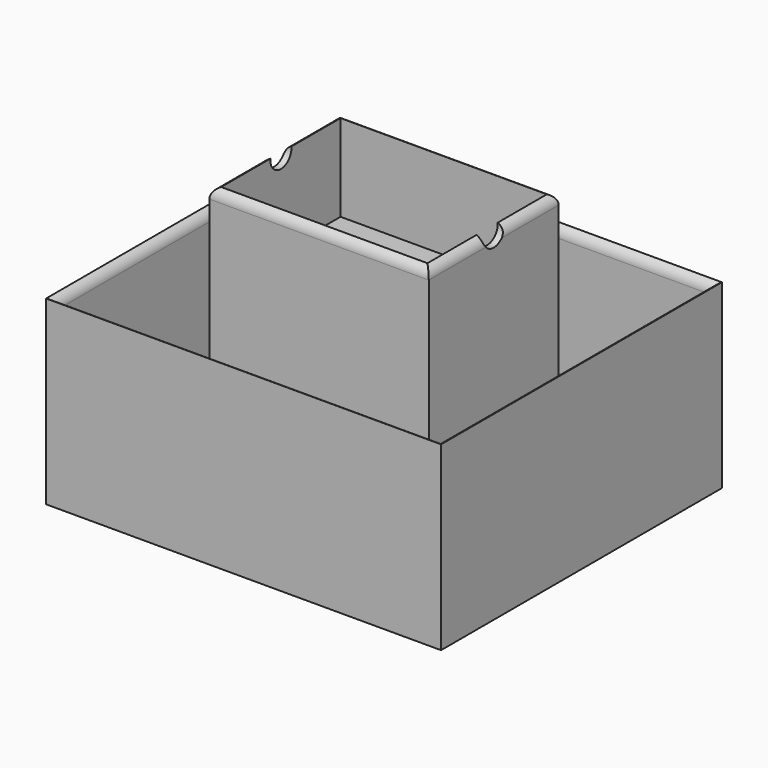
from build123d import *

# Parameters (mm, degrees)
F0_W          = 180
F0_H          = 160
F1_DEPTH      = 1
F2_W          = 10
F2_H          = 10
F3_DEPTH      = 50
F4_T          = 1
F4_T3_DEPTH   = 12
F4_T5_DEPTH   = 12
F4_T7_DEPTH   = 12
F4_T9_DEPTH   = 12
F5_W          = 180
F5_H          = 160
F6_DEPTH      = 3
F7_W          = 180
F7_H          = 160
F7_W_2        = 174
F7_H_2        = 154
F8_DEPTH      = 80
F9_W          = 100
F9_H          = 74
F10_DEPTH     = 120
F11_W         = 94
F11_H         = 68
F12_DEPTH     = 40
F14_T1_DEPTH  = 125
F14_T3_DEPTH  = 99
F14_T5_DEPTH  = 174
F14_T7_DEPTH  = 154
F14_T13_DEPTH = 166.5
F14_T19_DEPTH = 186.5
F14_T28_DEPTH = 166.5
F14_T34_DEPTH = 186.5
F14_T43_DEPTH = 186.5
F14_T49_DEPTH = 166.5
F14_T58_DEPTH = 166.5
F14_T64_DEPTH = 186.5
F15_R         = 6.0326848408
F16_DEPTH     = 500
F17_W         = 180
F17_H         = 160
F18_DEPTH     = 51
F13_W         = 94
F13_H         = 68
F19_DEPTH     = 80


# Not quite as in the source:
# - a fillet or chamfer that OpenCascade refuses, or shapes differently, is made with other operations: its cross-section is extruded or revolved along the edge and cut away or added
# - a shell that OpenCascade refuses in one call is made with other operations: the cavity is built on its own and cut out


with BuildPart() as f1:
    # F0 (on Top) → F1 (new body)
    with BuildSketch(Plane.XY):
        with Locations((-40, 0)):
            Rectangle(F0_W, F0_H)
    extrude(amount=F1_DEPTH)

    # F2 (on face) → F3 (join)
    with BuildSketch(Plane.XY.offset(1)):
        with Locations((-125, 75)):
            Rectangle(F2_W, F2_H)
        with Locations((45, 75)):
            Rectangle(F2_W, F2_H)
        with Locations((-125, -75)):
            Rectangle(F2_W, F2_H)
        with Locations((45, -75)):
            Rectangle(F2_W, F2_H)
    extrude(amount=F3_DEPTH)

    # F4: shell of thickness 1, made by hand


with BuildPart() as f4_core1:
    # F4_t2: copy of F1
    add(f1.part)

    # the walls: a layer under each face that stays
    f4_faces = [f4_core1.faces().sort_by_distance(p)[0] for p in [
        (44, 80, 49.3),
        (-124, -80, 49.3),
        (45, -75, 51),
        (45, -70, 26),
        (40, -75, 26),
        (-120, -75, 26),
        (-125, -70, 26),
        (-125, -75, 51),
        (-130, 74.6666666667, 49.3),
        (-125, 70, 26),
        (-125, 75, 51),
        (-120, 75, 26),
        (-40, 0, 1),
        (45, 70, 26),
        (40, 75, 26),
        (45, 75, 51),
        (50, -74.6666666667, 49.3),
    ]]
    thicken(f4_faces, amount=-F4_T, mode=Mode.SUBTRACT)

    # F4_s4 → F4_t3 (cut)
    with BuildSketch(Plane.YZ.offset(39)):
        Polygon((-69.99, 1.01), (-71, 1), (-71, 0), (-70, 0), align=None)
        Polygon((69.99, 1.01), (70, 0), (71, 0), (71, 1), align=None)
    extrude(amount=F4_T3_DEPTH, mode=Mode.SUBTRACT)

    # F4_s6 → F4_t5 (cut)
    with BuildSketch(Plane.XZ.offset(69)):
        Polygon((39.99, 1.01), (41, 1), (41, 0), (40, 0), align=None)
        Polygon((-119.99, 1.01), (-121, 1), (-121, 0), (-120, 0), align=None)
    extrude(amount=F4_T5_DEPTH, mode=Mode.SUBTRACT)

    # F4_s8 → F4_t7 (cut)
    with BuildSketch(Plane.YZ.offset(-131)):
        Polygon((-69.99, 1.01), (-71, 1), (-71, 0), (-70, 0), align=None)
        Polygon((69.99, 1.01), (71, 1), (71, 0), (70, 0), align=None)
    extrude(amount=F4_T7_DEPTH, mode=Mode.SUBTRACT)

    # F4_s10 → F4_t9 (cut)
    with BuildSketch(Plane.XZ.offset(-81)):
        Polygon((-119.99, 1.01), (-121, 1), (-121, 0), (-120, 0), align=None)
        Polygon((39.99, 1.01), (40, 0), (41, 0), (41, 1), align=None)
    extrude(amount=F4_T9_DEPTH, mode=Mode.SUBTRACT)


with BuildPart() as f1_1:
    add(f1.part)

    # what is left inside the walls is the cavity
    f4_cavity = [f4_core1.part.solids().sort_by_distance(p)[0] for p in [
        (45, 78.99, 33.333333),
        (-125, 78.99, 33.333333),
        (48.99, -75, 33.333333),
        (-123.666667, -71.01, 25),
    ]]
    add(f4_cavity, mode=Mode.SUBTRACT)

    # F5 (on face) → F6 (join)
    with BuildSketch(Plane.XY.offset(51)):
        with Locations((-40, 0)):
            Rectangle(F5_W, F5_H)
    extrude(amount=F6_DEPTH)

    # F7 (on face) → F8 (join)
    with BuildSketch(Plane.XY.offset(54)):
        with Locations((-40, 0)):
            Rectangle(F7_W, F7_H)
        with Locations((-40, 0)):
            Rectangle(F7_W_2, F7_H_2, mode=Mode.SUBTRACT)
    extrude(amount=F8_DEPTH)

    # F9 (on face) → F10 (join)
    with BuildSketch(Plane.XY.offset(54)):
        with Locations((-40, 0)):
            Rectangle(F9_W, F9_H)
    extrude(amount=F10_DEPTH)

    # F11 (on face) → F12 (cut)
    with BuildSketch(Plane.XY.offset(174)):
        with Locations((-40, 0)):
            Rectangle(F11_W, F11_H)
    extrude(amount=-F12_DEPTH, mode=Mode.SUBTRACT)

    # F14: fillet of radius 5 on 8 edges, made by hand

    # F14_s2 → F14_t1 (cut)
    with BuildSketch(Plane.YZ.offset(-102.5)):
        with BuildLine():
            ThreePointArc((-37, 169), (-35.5355339059, 172.5355339059), (-32, 174))
            Line((-32, 174), (-37, 174))
            Line((-37, 174), (-37, 169))
        make_face()
        with BuildLine():
            ThreePointArc((37, 169), (35.5355339059, 172.5355339059), (32, 174))
            Line((32, 174), (37, 174))
            Line((37, 174), (37, 169))
        make_face()
    extrude(amount=F14_T1_DEPTH, mode=Mode.SUBTRACT)

    # F14_s4 → F14_t3 (cut)
    with BuildSketch(Plane.XZ.offset(-49.5)):
        with BuildLine():
            ThreePointArc((-90, 169), (-88.5355339059, 172.5355339059), (-85, 174))
            Line((-85, 174), (-90, 174))
            Line((-90, 174), (-90, 169))
        make_face()
        with BuildLine():
            ThreePointArc((10, 169), (8.5355339059, 172.5355339059), (5, 174))
            Line((5, 174), (10, 174))
            Line((10, 174), (10, 169))
        make_face()
    extrude(amount=F14_T3_DEPTH, mode=Mode.SUBTRACT)

    # F14_s6 → F14_t5 (cut)
    with BuildSketch(Plane.YZ.offset(-127)):
        with BuildLine():
            ThreePointArc((-82, 134), (-78.4644660941, 132.5355339059), (-77, 129))
            Line((-77, 129), (-77, 134))
            Line((-77, 134), (-82, 134))
        make_face()
        with BuildLine():
            ThreePointArc((82, 134), (78.4644660941, 132.5355339059), (77, 129))
            Line((77, 129), (77, 134))
            Line((77, 134), (82, 134))
        make_face()
    extrude(amount=F14_T5_DEPTH, mode=Mode.SUBTRACT)

    # F14_s8 → F14_t7 (cut)
    with BuildSketch(Plane.XZ.offset(-77)):
        with BuildLine():
            ThreePointArc((52, 134), (48.4644660941, 132.5355339059), (47, 129))
            Line((47, 129), (47, 134))
            Line((47, 134), (52, 134))
        make_face()
        with BuildLine():
            ThreePointArc((-132, 134), (-128.4644660941, 132.5355339059), (-127, 129))
            Line((-127, 129), (-127, 134))
            Line((-127, 134), (-132, 134))
        make_face()
    extrude(amount=F14_T7_DEPTH, mode=Mode.SUBTRACT)


with BuildPart() as f14_tool11:
    # F14_s12 → F14_t13 (new body)
    with BuildSketch(Plane.XZ.offset(-77)):
        with BuildLine():
            ThreePointArc((52, 134), (48.4644660941, 132.5355339059), (47, 129))
            Line((47, 129), (47, 134))
            Line((47, 134), (52, 134))
        make_face()
    extrude(amount=F14_T13_DEPTH)

    split(bisect_by=Plane.YZ.offset(50), keep=Keep.BOTTOM)

    split(bisect_by=Plane.XZ.offset(80), keep=Keep.BOTTOM)

    split(bisect_by=Plane.XZ.offset(77), keep=Keep.TOP)


with BuildPart() as f14_tool17:
    # F14_s18 → F14_t19 (new body)
    with BuildSketch(Plane.YZ.offset(59.5)):
        with BuildLine():
            ThreePointArc((-82, 134), (-78.4644660941, 132.5355339059), (-77, 129))
            Line((-77, 129), (-77, 134))
            Line((-77, 134), (-82, 134))
        make_face()
    extrude(amount=-F14_T19_DEPTH)

    split(bisect_by=Plane.YZ.offset(50), keep=Keep.BOTTOM)

    split(bisect_by=Plane.XZ.offset(80), keep=Keep.BOTTOM)

    split(bisect_by=Plane.YZ.offset(47), keep=Keep.TOP)


with BuildPart() as f14_tool11_1:
    add(f14_tool11.part)

    # F14_t23: intersect F14_tool17
    add(f14_tool17.part, mode=Mode.INTERSECT)


with BuildPart() as f1_2:
    add(f1_1.part)

    # F14_t9: cut F14_tool11
    add(f14_tool11_1.part, mode=Mode.SUBTRACT)


with BuildPart() as f14_tool26:
    # F14_s27 → F14_t28 (new body)
    with BuildSketch(Plane.XZ.offset(89.5)):
        with BuildLine():
            ThreePointArc((-132, 134), (-128.4644660941, 132.5355339059), (-127, 129))
            Line((-127, 129), (-127, 134))
            Line((-127, 134), (-132, 134))
        make_face()
    extrude(amount=-F14_T28_DEPTH)

    split(bisect_by=Plane.YZ.offset(-130), keep=Keep.TOP)

    split(bisect_by=Plane.XZ.offset(80), keep=Keep.BOTTOM)

    split(bisect_by=Plane.XZ.offset(77), keep=Keep.TOP)


with BuildPart() as f14_tool32:
    # F14_s33 → F14_t34 (new body)
    with BuildSketch(Plane.YZ.offset(47)):
        with BuildLine():
            ThreePointArc((-82, 134), (-78.4644660941, 132.5355339059), (-77, 129))
            Line((-77, 129), (-77, 134))
            Line((-77, 134), (-82, 134))
        make_face()
    extrude(amount=-F14_T34_DEPTH)

    split(bisect_by=Plane.YZ.offset(-130), keep=Keep.TOP)

    split(bisect_by=Plane.XZ.offset(80), keep=Keep.BOTTOM)

    split(bisect_by=Plane.YZ.offset(-127), keep=Keep.BOTTOM)


with BuildPart() as f14_tool26_1:
    add(f14_tool26.part)

    # F14_t38: intersect F14_tool32
    add(f14_tool32.part, mode=Mode.INTERSECT)


with BuildPart() as f1_3:
    add(f1_2.part)

    # F14_t24: cut F14_tool26
    add(f14_tool26_1.part, mode=Mode.SUBTRACT)


with BuildPart() as f14_tool41:
    # F14_s42 → F14_t43 (new body)
    with BuildSketch(Plane.YZ.offset(-127)):
        with BuildLine():
            ThreePointArc((82, 134), (78.4644660941, 132.5355339059), (77, 129))
            Line((77, 129), (77, 134))
            Line((77, 134), (82, 134))
        make_face()
    extrude(amount=F14_T43_DEPTH)

    split(bisect_by=Plane.XZ.offset(-80), keep=Keep.TOP)

    split(bisect_by=Plane.YZ.offset(50), keep=Keep.BOTTOM)

    split(bisect_by=Plane.YZ.offset(47), keep=Keep.TOP)


with BuildPart() as f14_tool47:
    # F14_s48 → F14_t49 (new body)
    with BuildSketch(Plane.XZ.offset(-89.5)):
        with BuildLine():
            ThreePointArc((52, 134), (48.4644660941, 132.5355339059), (47, 129))
            Line((47, 129), (47, 134))
            Line((47, 134), (52, 134))
        make_face()
    extrude(amount=F14_T49_DEPTH)

    split(bisect_by=Plane.XZ.offset(-80), keep=Keep.TOP)

    split(bisect_by=Plane.YZ.offset(50), keep=Keep.BOTTOM)

    split(bisect_by=Plane.XZ.offset(-77), keep=Keep.BOTTOM)


with BuildPart() as f14_tool41_1:
    add(f14_tool41.part)

    # F14_t53: intersect F14_tool47
    add(f14_tool47.part, mode=Mode.INTERSECT)


with BuildPart() as f1_4:
    add(f1_3.part)

    # F14_t39: cut F14_tool41
    add(f14_tool41_1.part, mode=Mode.SUBTRACT)


with BuildPart() as f14_tool56:
    # F14_s57 → F14_t58 (new body)
    with BuildSketch(Plane.XZ.offset(77)):
        with BuildLine():
            ThreePointArc((-132, 134), (-128.4644660941, 132.5355339059), (-127, 129))
            Line((-127, 129), (-127, 134))
            Line((-127, 134), (-132, 134))
        make_face()
    extrude(amount=-F14_T58_DEPTH)

    split(bisect_by=Plane.XZ.offset(-80), keep=Keep.TOP)

    split(bisect_by=Plane.YZ.offset(-130), keep=Keep.TOP)

    split(bisect_by=Plane.XZ.offset(-77), keep=Keep.BOTTOM)


with BuildPart() as f14_tool62:
    # F14_s63 → F14_t64 (new body)
    with BuildSketch(Plane.YZ.offset(-139.5)):
        with BuildLine():
            ThreePointArc((82, 134), (78.4644660941, 132.5355339059), (77, 129))
            Line((77, 129), (77, 134))
            Line((77, 134), (82, 134))
        make_face()
    extrude(amount=F14_T64_DEPTH)

    split(bisect_by=Plane.XZ.offset(-80), keep=Keep.TOP)

    split(bisect_by=Plane.YZ.offset(-130), keep=Keep.TOP)

    split(bisect_by=Plane.YZ.offset(-127), keep=Keep.BOTTOM)


with BuildPart() as f14_tool56_1:
    add(f14_tool56.part)

    # F14_t68: intersect F14_tool62
    add(f14_tool62.part, mode=Mode.INTERSECT)


with BuildPart() as f1_5:
    add(f1_4.part)

    # F14_t54: cut F14_tool56
    add(f14_tool56_1.part, mode=Mode.SUBTRACT)

    # F15 (on face) → F16 (cut)
    with BuildSketch(Plane.YZ.offset(10)):
        with Locations((0, 173)):
            Circle(F15_R)
    extrude(amount=-F16_DEPTH, mode=Mode.SUBTRACT)

    # F17 (on face) → F18 (cut)
    with BuildSketch(Plane(origin=(0, 0, 0), x_dir=(1, 0, 0), z_dir=(0, 0, -1))):
        with Locations((-40, 0)):
            Rectangle(F17_W, F17_H)
    extrude(amount=-F18_DEPTH, mode=Mode.SUBTRACT)

    # F13 (on face) → F19 (cut)
    with BuildSketch(Plane(origin=(0, 0, 51), x_dir=(1, 0, 0), z_dir=(0, 0, -1))):
        with Locations((-40, 0)):
            Rectangle(F13_W, F13_H)
    extrude(amount=-F19_DEPTH, mode=Mode.SUBTRACT)


solid = f1_5.part
